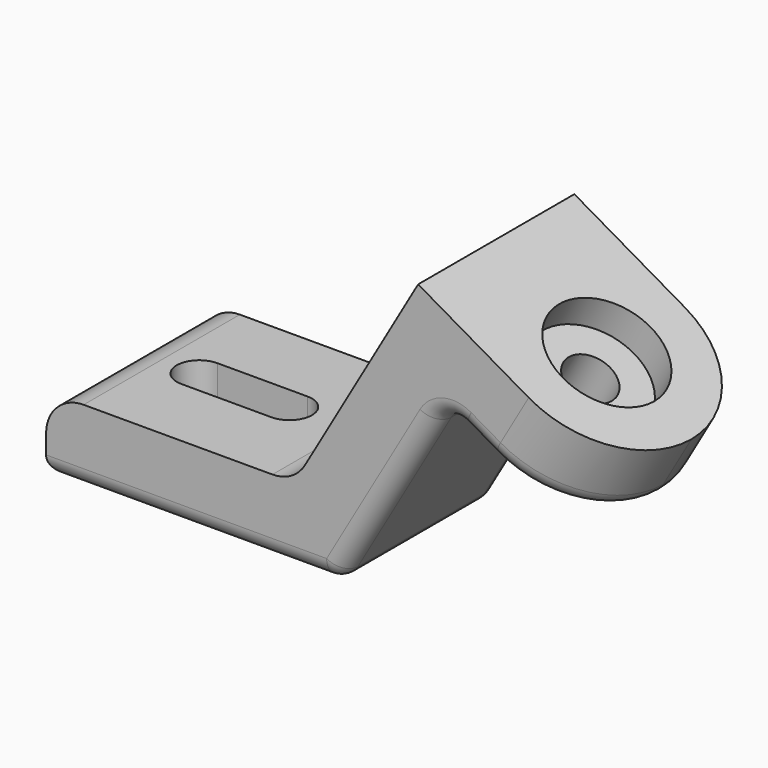
from build123d import *

# Parameters (mm, degrees)
F1_DEPTH    = 13
F3_DEPTH    = 10.001
F4_R        = 5
F5_R        = 2.5
F6_T1_DEPTH = 42.5
F6_T4_ANGLE = 90
F6_T6_ANGLE = 90
F7_R        = 3.3
F8_DEPTH    = 58.201
F7_R_2      = 7.3
F10_DEPTH   = 4.4


# Not quite as in the source:
# - a fillet or chamfer that OpenCascade refuses, or shapes differently, is made with other operations: its cross-section is extruded or revolved along the edge and cut away or added


with BuildPart() as f1:
    # F0 (on Front) → F1 (new body, symmetric)
    with BuildSketch(Plane.XZ):
        Polygon((0, 10), (0, 0), (38.8, 0), (53.2, 24.941531629), (70.5205080757, 14.941531629), (75.5205080757, 23.6017856668), (49.5397459622, 38.6017856668), (33.0264973081, 10), align=None)
    extrude(amount=F1_DEPTH, both=True)

    # F2 (on face) → F3 (cut, through all)
    with BuildSketch(Plane.XY.offset(10)):
        with BuildLine():
            ThreePointArc((10, 3), (7, 0), (10, -3))
            Line((10, -3), (22, -3))
            ThreePointArc((22, -3), (25, 0), (22, 3))
            Line((22, 3), (10, 3))
        make_face()
    extrude(amount=-F3_DEPTH, mode=Mode.SUBTRACT)

    # F4
    f4_edges = [f1.edges().sort_by_distance(p)[0] for p in [
        (0, 0, 10),
        (33.026497, 0, 10),
    ]]
    fillet(f4_edges, radius=F4_R)

    # F5
    f5_edges = [f1.edges().sort_by_distance(p)[0] for p in [
        (0, 0, 0),
        (19.4, -13, 0),
        (19.4, 13, 0),
        (38.8, 0, 0),
        (46, -13, 12.470766),
        (46, 13, 12.470766),
        (53.2, 0, 24.941532),
        (61.860254, -13, 19.941532),
        (61.860254, 13, 19.941532),
        (70.520508, 0, 14.941532),
    ]]
    fillet(f5_edges, radius=F5_R)

    # F6: fillet of radius 13 on 2 edges, made by hand

    # F6_s2 → F6_t1 (cut)
    with BuildSketch(Plane(origin=(24.1, 0, 41.7424244624), x_dir=(0, 1, 0), z_dir=(0.5, 0, 0.8660254038))):
        with BuildLine():
            ThreePointArc((-13, -40.6017856668), (-9.1923881554, -49.7941738223), (0, -53.6017856668))
            Line((0, -53.6017856668), (-13, -53.6017856668))
            Line((-13, -53.6017856668), (-13, -40.6017856668))
        make_face()
        with BuildLine():
            ThreePointArc((13, -40.6017856668), (9.1923881554, -49.7941738223), (0, -53.6017856668))
            Line((0, -53.6017856668), (13, -53.6017856668))
            Line((13, -53.6017856668), (13, -40.6017856668))
        make_face()
    extrude(amount=F6_T1_DEPTH, mode=Mode.SUBTRACT)

    # F6_s3 → F6_t4 (revolve, cut)
    with BuildSketch(Plane(origin=(35.1621778265, 0, -20.3008928334), x_dir=(0, 1, 0), z_dir=(-0.8660254038, 0, 0.5))):
        with BuildLine():
            ThreePointArc((10.5, -48.2), (12.267766953, -48.932233047), (13, -50.7))
            Line((13, -50.7), (13, -48.2))
            Line((13, -48.2), (10.5, -48.2))
        make_face()
    revolve(axis=Axis((59.2621778265, 0, 21.441531629), (-0.5, 0, -0.8660254038)), revolution_arc=F6_T4_ANGLE, mode=Mode.SUBTRACT)

    # F6_s5 → F6_t6 (revolve, cut)
    with BuildSketch(Plane.XZ):
        with BuildLine():
            ThreePointArc((68.3554445662, 16.191531629), (70.252492179, 15.9417805727), (71.7705080757, 17.1065951385))
            Line((71.7705080757, 17.1065951385), (70.5205080757, 14.941531629))
            Line((70.5205080757, 14.941531629), (68.3554445662, 16.191531629))
        make_face()
    revolve(axis=Axis((59.2621778265, 0, 21.441531629), (-0.5, 0, -0.8660254038)), revolution_arc=F6_T6_ANGLE, mode=Mode.SUBTRACT)

    # F7 (on face) → F8 (cut, through all)
    with BuildSketch(Plane(origin=(29.1, 0, 50.4026785003), x_dir=(0.8660254038, 0, -0.5), z_dir=(0.5, 0, 0.8660254038))):
        with Locations((40.6017856668, 0)):
            Circle(F7_R)
    extrude(amount=-F8_DEPTH, mode=Mode.SUBTRACT)

    # F7 (on face) → F10 (cut)
    with BuildSketch(Plane(origin=(29.1, 0, 50.4026785003), x_dir=(0.8660254038, 0, -0.5), z_dir=(0.5, 0, 0.8660254038))):
        with Locations((40.6017856668, 0)):
            Circle(F7_R_2)
        with Locations((40.6017856668, 0)):
            Circle(F7_R, mode=Mode.SUBTRACT)
    extrude(amount=-F10_DEPTH, mode=Mode.SUBTRACT)


solid = f1.part
